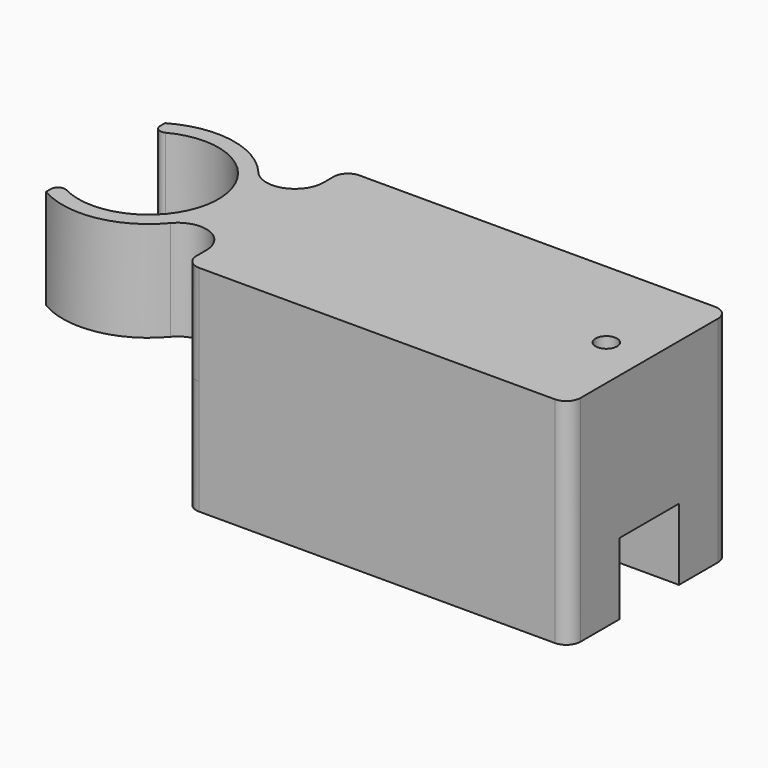
from build123d import *

# Parameters (mm, degrees)
F0_W         = 38
F0_H         = 14
F1_DEPTH     = 15
F2_R         = 4.8895
F3_DEPTH     = 15.001
F4_W         = 30.8590809897
F4_H         = 5.2
F5_DEPTH     = 5
F7_DEPTH     = 15.001
F8_W         = 13.0838444641
F8_H         = 13.9913465828
F9_DEPTH     = 8
F11_R        = 0.75
F12_DEPTH    = 15.001
F13_R        = 0.5
F14_T1_DEPTH = 9.498744071
F14_T3_DEPTH = 10.5
F14_T5_DEPTH = 20


# Not quite as in the source:
# - a fillet or chamfer that OpenCascade refuses, or shapes differently, is made with other operations: its cross-section is extruded or revolved along the edge and cut away or added


with BuildPart() as f1:
    # F0 (on Top) → F1 (new body)
    with BuildSketch(Plane.XY):
        with Locations((19, 7)):
            Rectangle(F0_W, F0_H)
    extrude(amount=F1_DEPTH)

    # F2 (on face) → F3 (cut, through all)
    with BuildSketch(Plane.XY.offset(15)):
        with Locations((3, 7)):
            Circle(F2_R)
    extrude(amount=-F3_DEPTH, mode=Mode.SUBTRACT)

    # F4 (on face) → F5 (cut)
    with BuildSketch(Plane(origin=(0, 0, 0), x_dir=(1, 0, 0), z_dir=(0, 0, -1))):
        with Locations((22.5704595052, -7)):
            Rectangle(F4_W, F4_H)
    extrude(amount=-F5_DEPTH, mode=Mode.SUBTRACT)

    # F6 (on face) → F7 (cut, through all)
    with BuildSketch(Plane.XY.offset(15)):
        with BuildLine():
            ThreePointArc((7.60725, 3.1564017591), (4.0503160688, 1.0926455874), (0, 1.8038475773))
            Line((0, 1.8038475773), (0, 0))
            Line((0, 0), (11.143, 0))
            Line((11.143, 0), (11.1420263596, 1.9376011727))
            ThreePointArc((11.1420263596, 1.9376011727), (9.7949393865, 3.7659627841), (7.60725, 3.1564017591))
        make_face()
        with BuildLine():
            ThreePointArc((0, 12.1961524227), (4.0503160688, 12.9073544126), (7.60725, 10.8435982409))
            ThreePointArc((7.60725, 10.8435982409), (9.7949393865, 10.2340372159), (11.1420263596, 12.0623988273))
            Line((11.1420263596, 12.0623988273), (11.1420263596, 14))
            Line((11.1420263596, 14), (0, 14))
            Line((0, 14), (0, 12.1961524227))
        make_face()
    extrude(amount=-F7_DEPTH, mode=Mode.SUBTRACT)

    # F8 (on face) → F9 (cut)
    with BuildSketch(Plane(origin=(0, 0, 0), x_dir=(1, 0, 0), z_dir=(0, 0, -1))):
        with Locations((4.6010777679, -6.9956732914)):
            Rectangle(F8_W, F8_H)
    extrude(amount=-F9_DEPTH, mode=Mode.SUBTRACT)

    # F11 (on face) → F12 (cut, through all)
    with BuildSketch(Plane.XY.offset(15)):
        with Locations((35, 7)):
            Circle(F11_R)
    extrude(amount=-F12_DEPTH, mode=Mode.SUBTRACT)

    # F13
    f13_edges = [f1.edges().sort_by_distance(p)[0] for p in [
        (0, 10.860986, 11.5),
        (0, 3.139014, 11.5),
    ]]
    fillet(f13_edges, radius=F13_R)

    # F14: fillet of radius 1 on 5 edges, made by hand

    # F14_s2 → F14_t1 (cut)
    with BuildSketch(Plane.XY.offset(8)):
        with BuildLine():
            ThreePointArc((11.1424977547, 0.9994975022), (11.4355685293, 0.2927155813), (12.1424976284, 0))
            Line((12.1424976284, 0), (11.143, 0))
            Line((11.143, 0), (11.1424977547, 0.9994975022))
        make_face()
    extrude(amount=F14_T1_DEPTH, mode=Mode.SUBTRACT)

    # F14_s4 → F14_t3 (cut)
    with BuildSketch(Plane.XY.offset(-2.5)):
        with BuildLine():
            ThreePointArc((11.143, 1), (11.4358932188, 0.2928932188), (12.143, 0))
            Line((12.143, 0), (11.143, 0))
            Line((11.143, 0), (11.143, 1))
        make_face()
    extrude(amount=F14_T3_DEPTH, mode=Mode.SUBTRACT)

    # F14_s6 → F14_t5 (cut)
    with BuildSketch(Plane.XY.offset(-2.5)):
        with BuildLine():
            ThreePointArc((37, 0), (37.7071067812, 0.2928932188), (38, 1))
            Line((38, 1), (38, 0))
            Line((38, 0), (37, 0))
        make_face()
        with BuildLine():
            ThreePointArc((11.1420263596, 13), (11.4349195784, 13.7071067812), (12.1420263596, 14))
            Line((12.1420263596, 14), (11.1420263596, 14))
            Line((11.1420263596, 14), (11.1420263596, 13))
        make_face()
        with BuildLine():
            ThreePointArc((38, 13), (37.7071067812, 13.7071067812), (37, 14))
            Line((37, 14), (38, 14))
            Line((38, 14), (38, 13))
        make_face()
    extrude(amount=F14_T5_DEPTH, mode=Mode.SUBTRACT)


solid = f1.part
